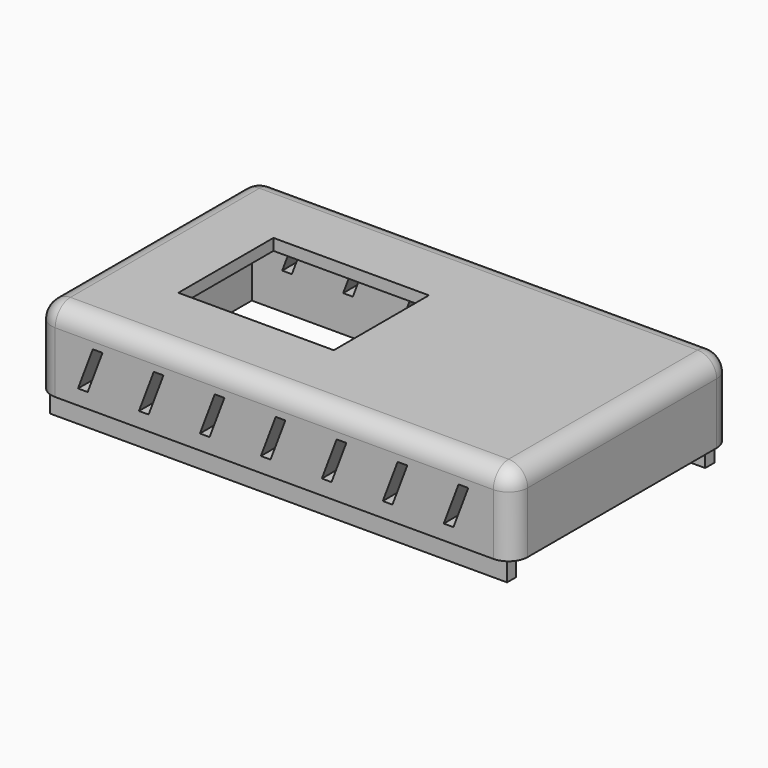
from build123d import *

# Parameters (mm, degrees)
F1_DEPTH  = 2.8
F0_W      = 62.5
F0_H      = 36
F2_DEPTH  = 9
F3_W      = 36
F3_H      = 1.5
F4_DEPTH  = 62.5
F5_R      = 2.5
F6_DEPTH  = 1
F9_W      = 20.4
F9_H      = 15.6
F10_DEPTH = 13.301
F12_DEPTH = 50


# Not quite as in the source:
# - a feature names something its author has since deleted; it is built from what else it names


with BuildPart() as f1:
    # F0 (on Top) → F1 (new body)
    with BuildSketch(Plane.XY):
        Polygon((29.8387005084, 17), (-30.1612994916, 17), (-30.1612994916, -17), (29.8387005084, -17), (29.8387005084, -15.5), (-28.6612994916, -15.5), (-28.6612994916, 15.5), (29.8387005084, 15.5), align=None)
    extrude(amount=-F1_DEPTH)

    # F0 (on Top) → F2 (join)
    with BuildSketch(Plane.XY):
        with Locations((0.0887005084, 0)):
            Rectangle(F0_W, F0_H)
        Polygon((-30.1612994916, -17), (-30.1612994916, 17), (29.8387005084, 17), (29.8387005084, 15.5), (29.8387005084, -15.5), (29.8387005084, -17), align=None, mode=Mode.SUBTRACT)
        Polygon((29.8387005084, 17), (-30.1612994916, 17), (-30.1612994916, -17), (29.8387005084, -17), (29.8387005084, -15.5), (-28.6612994916, -15.5), (-28.6612994916, 15.5), (29.8387005084, 15.5), align=None)
    extrude(amount=F2_DEPTH)

    # F3 (on face) → F4 (join, through all)
    with BuildSketch(Plane.YZ.offset(31.3387005084)):
        with Locations((0, 9.75)):
            Rectangle(F3_W, F3_H)
    extrude(amount=-F4_DEPTH)

    # F5
    f5_edges = [f1.edges().sort_by_distance(p)[0] for p in [
        (31.338701, 0, 10.5),
        (0.088701, -18, 10.5),
        (31.338701, -18, 5.25),
        (31.338701, 18, 5.25),
        (0.088701, 18, 10.5),
        (-31.161299, 18, 5.25),
        (-31.161299, 0, 10.5),
        (-31.161299, -18, 5.25),
    ]]
    fillet(f5_edges, radius=F5_R)

    # F6 (cut): a face of the model
    f6_faces = [f1.faces().sort_by_distance(p)[0] for p in [
        (-28.6612994916, 0, 3.1),
    ]]
    extrude(f6_faces, amount=-F6_DEPTH, mode=Mode.SUBTRACT)

    # F9 (on face) → F10 (cut, through all)
    with BuildSketch(Plane.XY.offset(10.5)):
        with Locations((-10.4612994916, 0)):
            Rectangle(F9_W, F9_H)
    extrude(amount=-F10_DEPTH, mode=Mode.SUBTRACT)

    # F11 (on face) → F12 (cut)
    with BuildSketch(Plane.XZ.offset(18)):
        Polygon((-23.7249415368, 7.122464478), (-25.6706383079, 1.9621371757), (-24.4017057121, 1.9621371757), (-22.4560089409, 7.122464478), align=None)
        Polygon((-15.7249415368, 7.122464478), (-17.6706383079, 1.9621371757), (-16.4017057121, 1.9621371757), (-14.4560089409, 7.122464478), align=None)
        Polygon((-7.7249415368, 7.122464478), (-9.6706383079, 1.9621371757), (-8.4017057121, 1.9621371757), (-6.4560089409, 7.122464478), align=None)
        Polygon((0.2750584632, 7.122464478), (-1.6706383079, 1.9621371757), (-0.4017057121, 1.9621371757), (1.5439910591, 7.122464478), align=None)
        Polygon((8.2750584632, 7.122464478), (6.3293616921, 1.9621371757), (7.5982942879, 1.9621371757), (9.5439910591, 7.122464478), align=None)
        Polygon((16.2750584632, 7.122464478), (14.3293616921, 1.9621371757), (15.5982942879, 1.9621371757), (17.5439910591, 7.122464478), align=None)
        Polygon((24.2750584632, 7.122464478), (22.3293616921, 1.9621371757), (23.5982942879, 1.9621371757), (25.5439910591, 7.122464478), align=None)
    extrude(amount=-F12_DEPTH, mode=Mode.SUBTRACT)


solid = f1.part
